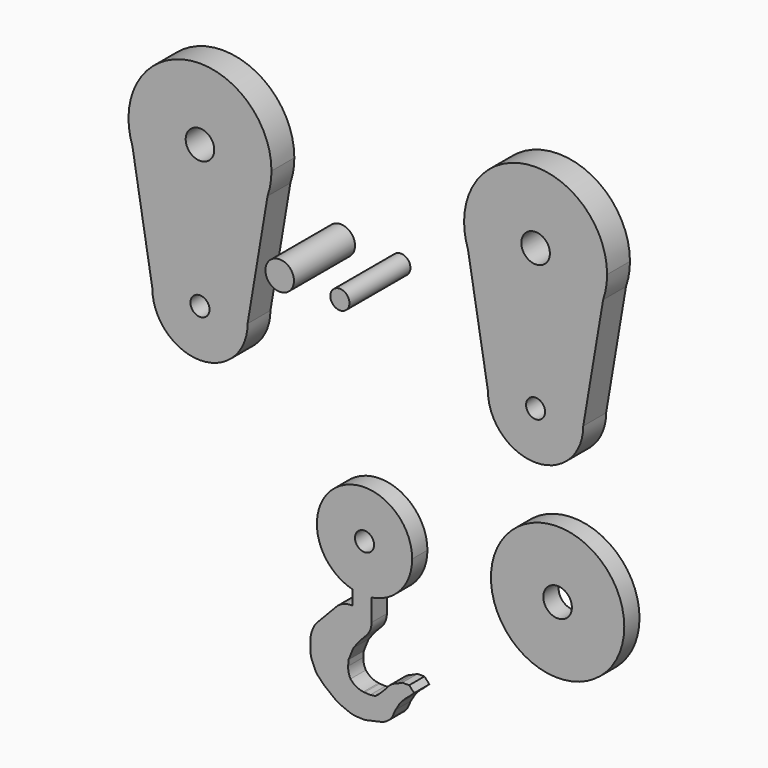
from build123d import *

# Parameters (mm, degrees)
F1_DEPTH     = 7.62
F2_D         = 5.08
F4_DEPTH     = 7.62
F5_D         = 7.62
F6_D         = 7.62
F7_D         = 5.08
F9_DEPTH     = 5.08
F10_T1_DEPTH = 15.6779412076
F11_R        = 5.08
F12_R        = 5.08
F13_R        = 5.08
F14_T1_DEPTH = 5.08
F14_F3_R     = 5.08
F15_R        = 5.08
F16_D        = 5.08
F17_R        = 17.7680692018
F18_DEPTH    = 5.08
F19_D        = 7.62
F20_R        = 3.8094085712
F21_DEPTH    = 20.32
F20_R_2      = 2.5450619433


# Not quite as in the source:
# - a fillet or chamfer that OpenCascade refuses, or shapes differently, is made with other operations: its cross-section is extruded or revolved along the edge and cut away or added


with BuildPart() as f1:
    # F0 (on Front) → F1 (new body)
    with BuildSketch(Plane.XZ):
        with BuildLine():
            Line((-23.8130350034, 31.6741682533), (-22.7673095988, 37.8994755447))
            ThreePointArc((-22.7673095988, 37.8994755447), (-41.8201088905, 56.9522748364), (-60.8729081823, 37.8994755447))
            Line((-60.8729081823, 37.8994755447), (-59.8271827777, 31.6741682533))
            ThreePointArc((-59.8271827777, 31.6741682533), (-41.8201088905, 18.846676253), (-23.8130350034, 31.6741682533))
        make_face()
        with BuildLine():
            ThreePointArc((-23.8130350034, 31.6741682533), (-23.0305595951, 34.7432122281), (-22.7673095988, 37.8994755447))
            Line((-22.7673095988, 37.8994755447), (-23.8130350034, 31.6741682533))
        make_face()
        with BuildLine():
            Line((-59.8271827777, 31.6741682533), (-60.8729081823, 37.8994755447))
            ThreePointArc((-60.8729081823, 37.8994755447), (-60.609658186, 34.7432122281), (-59.8271827777, 31.6741682533))
        make_face()
        with BuildLine():
            Line((-29.1336530644, 0), (-23.8130350034, 31.6741682533))
            ThreePointArc((-23.8130350034, 31.6741682533), (-41.8201088905, 18.846676253), (-59.8271827777, 31.6741682533))
            Line((-59.8271827777, 31.6741682533), (-54.5065647167, 0))
            ThreePointArc((-54.5065647167, 0), (-41.8201088905, 12.6864558261), (-29.1336530644, 0))
        make_face()
        with BuildLine():
            ThreePointArc((-54.5065647167, 0), (-41.8201088905, -12.6864558261), (-29.1336530644, 0))
            ThreePointArc((-29.1336530644, 0), (-41.8201088905, 12.6864558261), (-54.5065647167, 0))
        make_face()
    extrude(amount=F1_DEPTH)

    # F2 (through all)
    with Locations(Plane(origin=(0, 0, 0), x_dir=(1, 0, 0), z_dir=(0, 1, 0))):
        with Locations((-41.8201088905, 0)):
            Hole(F2_D / 2)

    # F5 (through all)
    with Locations(Plane(origin=(0, 0, 0), x_dir=(1, 0, 0), z_dir=(0, 1, 0))):
        with Locations((-41.8201088905, -37.8994755447)):
            Hole(F5_D / 2)


with BuildPart() as f4:
    # F3 (on Front) → F4 (new body)
    with BuildSketch(Plane.XZ):
        with BuildLine():
            Line((59.5282177794, 31.3490809442), (60.5857727855, 37.6090556383))
            ThreePointArc((60.5857727855, 37.6090556383), (41.5296927094, 56.6651357143), (22.4736126334, 37.6090556383))
            Line((22.4736126334, 37.6090556383), (23.5311676395, 31.3490809442))
            ThreePointArc((23.5311676395, 31.3490809442), (41.5296927094, 18.5529755623), (59.5282177794, 31.3490809442))
        make_face()
        with BuildLine():
            ThreePointArc((59.5282177794, 31.3490809442), (60.3195240398, 34.4347168977), (60.5857727855, 37.6090556383))
            Line((60.5857727855, 37.6090556383), (59.5282177794, 31.3490809442))
        make_face()
        with BuildLine():
            Line((23.5311676395, 31.3490809442), (22.4736126334, 37.6090556383))
            ThreePointArc((22.4736126334, 37.6090556383), (22.7398613791, 34.4347168977), (23.5311676395, 31.3490809442))
        make_face()
        with BuildLine():
            Line((54.2321296786, 0), (59.5282177794, 31.3490809442))
            ThreePointArc((59.5282177794, 31.3490809442), (41.5296927094, 18.5529755623), (23.5311676395, 31.3490809442))
            Line((23.5311676395, 31.3490809442), (28.8272557403, 0))
            ThreePointArc((28.8272557403, 0), (41.5296927094, 12.7024369691), (54.2321296786, 0))
        make_face()
        with BuildLine():
            ThreePointArc((28.8272557403, 0), (41.5296927094, -12.7024369691), (54.2321296786, 0))
            ThreePointArc((54.2321296786, 0), (41.5296927094, 12.7024369691), (28.8272557403, 0))
        make_face()
    extrude(amount=-F4_DEPTH)

    # F6 (through all)
    with Locations(Plane.XZ):
        with Locations((41.5296927094, 37.6090556383)):
            Hole(F6_D / 2)

    # F7 (through all)
    with Locations(Plane.XZ):
        with Locations((41.5296927094, 0)):
            Hole(F7_D / 2)


with BuildPart() as f9:
    # F8 (on Front) → F9 (new body)
    with BuildSketch(Plane.XZ):
        with BuildLine():
            ThreePointArc((1.8835700949, -55.1916896292), (9.6229496478, -50.9198456578), (12.699669381, -42.6324792206))
            ThreePointArc((12.699669381, -42.6324792206), (-7.7595267274, -32.5790545626), (-3.2174926052, -54.9178096486))
            ThreePointArc((-3.2174926052, -54.9178096486), (-0.6808743473, -55.3138834217), (1.8835700949, -55.1916896292))
        make_face()
        with BuildLine():
            ThreePointArc((1.8835700949, -55.1916896292), (-0.6808743473, -55.3138834217), (-3.2174926052, -54.9178096486))
            Line((-3.2174926052, -54.9178096486), (-3.2174926052, -58.7645881589))
            Line((-3.2174926052, -58.7645881589), (-5.4759941995, -58.7645881589))
            Line((-5.4759941995, -58.7645881589), (-7.29507301, -60.1794272661))
            Line((-7.29507301, -60.1794272661), (-13.2576106116, -66.4451420307))
            Line((-13.2576106116, -66.4451420307), (-14.369269833, -69.0727010369))
            Line((-14.369269833, -69.0727010369), (-14.369269833, -71.5992003679))
            Line((-14.369269833, -71.5992003679), (-14.369269833, -74.2267593741))
            Line((-14.369269833, -74.2267593741), (-12.8533700481, -77.7638554573))
            Line((-12.8533700481, -77.7638554573), (-10.6300516054, -79.9871757627))
            Line((-10.6300516054, -79.9871757627), (-7.1940133348, -82.7157944441))
            Line((-7.1940133348, -82.7157944441), (-3.2526752912, -84.3327566981))
            Line((-3.2526752912, -84.3327566981), (0, -84.5348760486))
            Line((0, -84.5348760486), (6.3480199315, -83.120033145))
            Line((6.3480199315, -83.120033145), (7.3586194776, -81.5030783415))
            Line((7.3586194776, -81.5030783415), (8.2681588829, -79.4818773866))
            Line((8.2681588829, -79.4818773866), (9.4808777794, -77.4606764317))
            Line((9.4808777794, -77.4606764317), (10.7946563512, -76.0458409786))
            Line((10.7946563512, -76.0458409786), (12.0688441613, -74.9925974282))
            Line((12.0688441613, -74.9925974282), (13.2200969383, -73.9235803485))
            Line((13.2200969383, -73.9235803485), (11.9063183665, -72.5087374449))
            Line((11.9063183665, -72.5087374449), (10.0872376934, -72.5087374449))
            Line((10.0872376934, -72.5087374449), (8.5713388398, -73.216162622))
            Line((8.5713388398, -73.216162622), (6.9543798454, -73.7214609981))
            Line((6.9543798454, -73.7214609981), (5.640600808, -75.4394754767))
            Line((5.640600808, -75.4394754767), (3.8215208333, -77.2585570812))
            Line((3.8215208333, -77.2585570812), (2.9119816609, -77.9659748077))
            Line((2.9119816609, -77.9659748077), (1.497142599, -78.1680941582))
            Line((1.497142599, -78.1680941582), (0, -78.067034483))
            Line((0, -78.067034483), (-2.6463153772, -77.7638554573))
            Line((-2.6463153772, -77.7638554573), (-4.4653946534, -75.0352367759))
            Line((-4.4653946534, -75.0352367759), (-4.2632748373, -71.8013197184))
            Line((-4.2632748373, -71.8013197184), (-2.949495567, -68.5674026608))
            Line((-2.949495567, -68.5674026608), (-1.2314763153, -66.3440823555))
            Line((-1.2314763153, -66.3440823555), (0.8931973609, -64.120400207))
            Line((0.8931973609, -64.120400207), (1.8835700949, -62.9080462995))
            Line((1.8835700949, -62.9080462995), (1.8835700949, -61.3925094736))
            Line((1.8835700949, -61.3925094736), (1.8835700949, -59.169189184))
            Line((1.8835700949, -59.169189184), (1.8835700949, -55.1916896292))
        make_face()
    extrude(amount=F9_DEPTH)

    # F10: fillet of radius 5.08 on 1 edges, made by hand

    # F10_s2 → F10_t1 (cut)
    with BuildSketch(Plane.XZ.offset(-5.2989706038)):
        with BuildLine():
            ThreePointArc((4.2791936374, -83.5811319179), (6.0156790125, -82.833698277), (7.3586194776, -81.5030783415))
            Line((7.3586194776, -81.5030783415), (6.3480199315, -83.120033145))
            Line((6.3480199315, -83.120033145), (4.2791936374, -83.5811319179))
        make_face()
    extrude(amount=F10_T1_DEPTH, mode=Mode.SUBTRACT)

    # F11
    f11_edges = [f9.edges().sort_by_distance(p)[0] for p in [
        (-3.252675, -2.54, -84.332757),
        (-7.194013, -2.54, -82.715794),
        (-10.630052, -2.54, -79.987176),
        (0, -2.54, -84.534876),
    ]]
    fillet(f11_edges, radius=F11_R)

    # F12
    f12_edges = [f9.edges().sort_by_distance(p)[0] for p in [
        (6.95438, -2.54, -73.721461),
    ]]
    fillet(f12_edges, radius=F12_R)

    # F13
    f13_edges = [f9.edges().sort_by_distance(p)[0] for p in [
        (-14.36927, -2.54, -74.226759),
        (-5.475994, -2.54, -58.764588),
    ]]
    fillet(f13_edges, radius=F13_R)

    # F14: fillet of radius 5.08 on 3 edges, made by hand

    # F14_s2 → F14_t1 (join)
    with BuildSketch(Plane.XZ):
        with BuildLine():
            ThreePointArc((-4.3585477158, -73.3256857753), (-4.1940364205, -74.9622378117), (-3.5152560014, -76.4604446322))
            Line((-3.5152560014, -76.4604446322), (-3.5997923091, -76.5168021755))
            Line((-3.5997923091, -76.5168021755), (-4.5689337341, -75.063090162))
            Line((-4.5689337341, -75.063090162), (-4.4599498578, -73.3193481414))
            Line((-4.4599498578, -73.3193481414), (-4.3585477158, -73.3256857753))
        make_face()
        with BuildLine():
            ThreePointArc((-3.9535608414, -75.8029874283), (-2.3752000359, -77.3200945031), (-0.3049608466, -78.0320961936))
            Line((-0.3049608466, -78.0320961936), (-0.3165251543, -78.1330359122))
            Line((-0.3165251543, -78.1330359122), (-2.7047067756, -77.8594303612))
            Line((-2.7047067756, -77.8594303612), (-4.0380971491, -75.8593449716))
            Line((-4.0380971491, -75.8593449716), (-3.9535608414, -75.8029874283))
        make_face()
    extrude(amount=F14_T1_DEPTH)

    # F14_f3
    f14_f3_edges = [f9.edges().sort_by_distance(p)[0] for p in [
        (1.8835700949, -2.54, -62.9080462995),
    ]]
    fillet(f14_f3_edges, radius=F14_F3_R)

    # F15
    f15_edges = [f9.edges().sort_by_distance(p)[0] for p in [
        (-13.257611, -2.54, -66.445142),
        (-14.36927, -2.54, -69.072701),
        (-12.85337, -2.54, -77.763855),
    ]]
    fillet(f15_edges, radius=F15_R)

    # F16 (through all)
    with Locations(Plane(origin=(0, 0, 0), x_dir=(1, 0, 0), z_dir=(0, 1, 0))):
        with Locations((0, 42.6324792206)):
            Hole(F16_D / 2)


with BuildPart() as f18:
    # F17 (on Front) → F18 (new body)
    with BuildSketch(Plane.XZ):
        with Locations((51.4584966004, -40.1577576995)):
            Circle(F17_R)
    extrude(amount=F18_DEPTH)

    # F19 (through all)
    with Locations(Plane(origin=(0, 0, 0), x_dir=(1, 0, 0), z_dir=(0, 1, 0))):
        with Locations((51.4584966004, 40.1577576995)):
            Hole(F19_D / 2)


with BuildPart() as f21:
    # F20 (on Front) → F21 (new body)
    with BuildSketch(Plane.XZ):
        with Locations((-10.4072010145, 22.5467532873)):
            Circle(F20_R)
    extrude(amount=F21_DEPTH)


with BuildPart() as f21b:
    # F20 (on Front) → F21, piece 2 (new body)
    with BuildSketch(Plane.XZ):
        with Locations((5.6285150349, 22.1340265125)):
            Circle(F20_R_2)
    extrude(amount=F21_DEPTH)


solid = Compound([f1.part, f4.part, f9.part, f18.part, f21.part, f21b.part])
